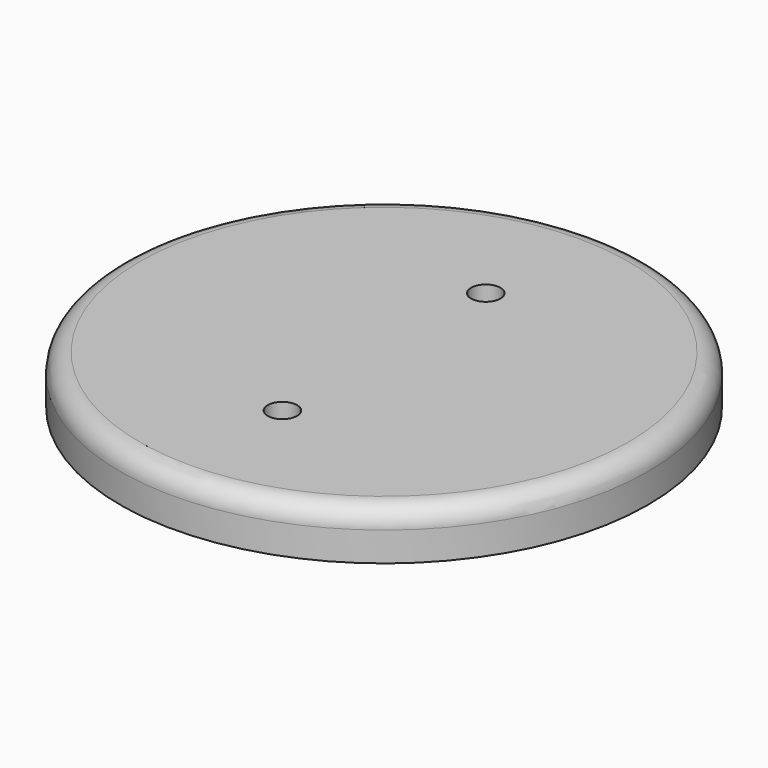
from build123d import *

# Parameters (mm, degrees)
F0_R     = 27
F1_DEPTH = 5
F2_R     = 2
F3_R     = 1.5
F4_DEPTH = 5.001


with BuildPart() as f1:
    # F0 (on Top) → F1 (new body)
    with BuildSketch(Plane.XY):
        Circle(F0_R)
    extrude(amount=F1_DEPTH)

    # F2
    f2_edges = [f1.edges().sort_by_distance(p)[0] for p in [
        (-27, 0, 5),
    ]]
    fillet(f2_edges, radius=F2_R)

    # F3 (on face) → F4 (cut, through all)
    with BuildSketch(Plane(origin=(0, 0, 0), x_dir=(1, 0, 0), z_dir=(0, 0, -1))):
        with Locations((0, 13)):
            Circle(F3_R)
        with Locations((0, -13)):
            Circle(F3_R)
    extrude(amount=-F4_DEPTH, mode=Mode.SUBTRACT)


solid = f1.part
